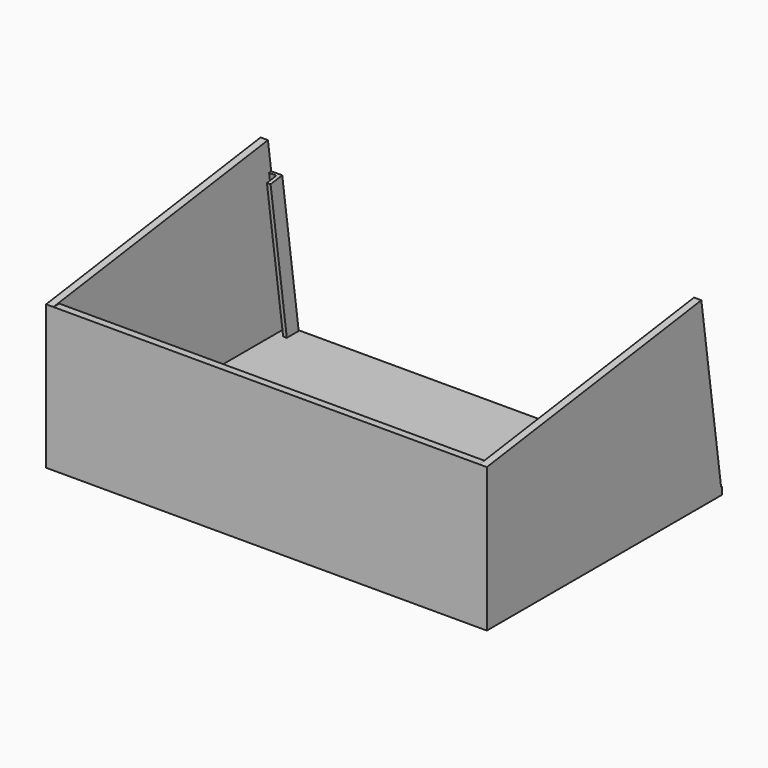
from build123d import *

# Parameters (mm, degrees)
F0_W      = 120
F0_H      = 80
F1_DEPTH  = 2
F3_DEPTH  = 2
F5_W      = 116
F5_H      = 37.1859224175
F6_DEPTH  = 2
F8_DEPTH  = 3
F9_W      = 1.9952932298
F9_H      = 3.2731545162
F10_REACH = 45.8542642129


with BuildPart() as f1:
    # F0 (on Top) → F1 (new body)
    with BuildSketch(Plane.XY):
        with Locations((0, 16.5011590771)):
            Rectangle(F0_W, F0_H)
    extrude(amount=F1_DEPTH)

    # F2 (on face) → F3 (join)
    with BuildSketch(Plane.YZ.offset(60)):
        Polygon((-23.4988409229, 2), (56.2183740699, 2), (49.5011590771, 49.5075751779), (-23.4988409229, 39.1859224175), align=None)
    extrude(amount=-F3_DEPTH)

    # F4: F1 across plane


with BuildPart() as f1_1:
    add(f1.part)
    add(f1.part.mirror(Plane.YZ))

    # F5 (on face) → F6 (join)
    with BuildSketch(Plane.XZ.offset(23.4988409229)):
        with Locations((0, 20.5929612087)):
            Rectangle(F5_W, F5_H)
    extrude(amount=-F6_DEPTH)

    # F7 (on face) → F8 (join)
    with BuildSketch(Plane.YZ.offset(-58)):
        Polygon((52.1785882537, 2), (56.2183740699, 2), (50.6183740699, 41.6060601424), (46.6577680557, 41.0460601424), align=None)
    extrude(amount=F8_DEPTH)

    f10_end = Plane(origin=(0.0757710305, 17.4568088596, 2), x_dir=(1, 0, 0), z_dir=(0, 0, 1))
    # F9 (on face) → F10 (cut, up to a plane its end follows)
    with BuildSketch(Plane(origin=(0, -4.7753622892, 33.7738010765), x_dir=(1, 0, 0), z_dir=(0, -0.14, 0.9901515036))):
        with Locations((-57.0023533851, 53.5812848711)):
            Rectangle(F9_W, F9_H)
    f10_long = extrude(amount=-F10_REACH, mode=Mode.PRIVATE)
    add(split(f10_long, bisect_by=f10_end, keep=Keep.TOP, mode=Mode.PRIVATE), mode=Mode.SUBTRACT)

    # F11: F1 across plane


with BuildPart() as f1_2:
    add(f1_1.part)
    add(f1_1.part.mirror(Plane.YZ))


solid = f1_2.part
